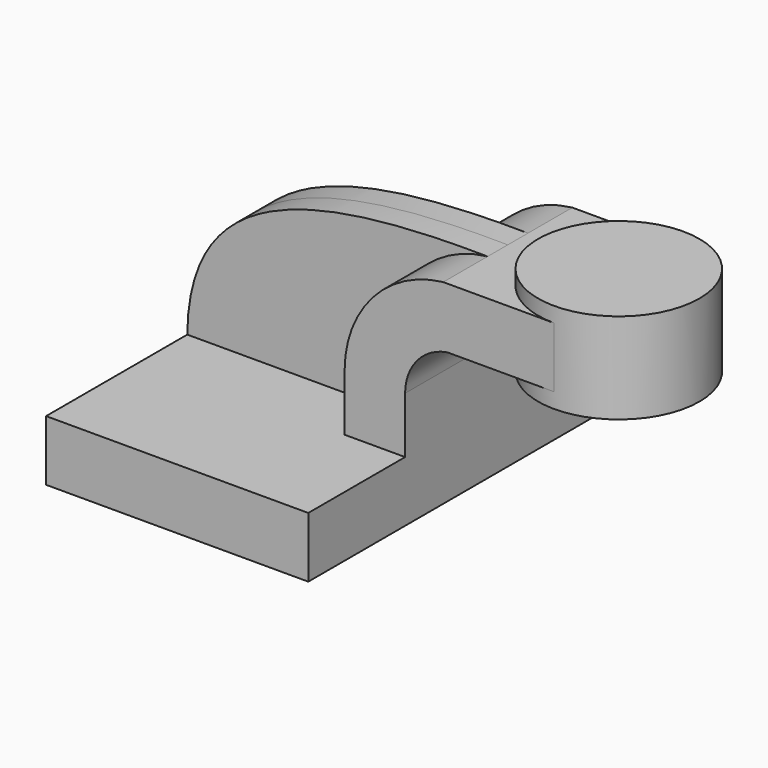
from build123d import *

# Parameters (mm, degrees)
F1_DEPTH = 63.5
F0_W     = 25.4
F0_H     = 19.05
F2_DEPTH = 25.4
F3_DEPTH = 7.9375


with BuildPart() as f1:
    # F0 (on Front) → F1 (new body, symmetric)
    with BuildSketch(Plane.XZ):
        Polygon((-41.275, 9.525), (-41.275, -9.525), (41.275, -9.525), (41.275, 9.525), (22.225, 9.525), align=None)
    extrude(amount=F1_DEPTH, both=True)

    # F0 (on Front) → F2 (join, symmetric)
    with BuildSketch(Plane.XZ):
        with Locations((75.5235318422, 52.4002)):
            Rectangle(F0_W, F0_H)
        with BuildLine():
            Line((22.225, 9.525), (41.275, 9.525))
            Line((41.275, 9.525), (41.275, 27.2153939429))
            ThreePointArc((41.275, 27.2153939429), (45.0386370244, 37.4784593657), (54.5449857479, 42.8752))
            Line((54.5449857479, 42.8752), (62.8235318422, 42.8752))
            Line((62.8235318422, 42.8752), (62.8235318422, 61.9252))
            Line((62.8235318422, 61.9252), (53.2789551181, 61.9252))
            ThreePointArc((53.2789551181, 61.9252), (31.1216321343, 50.5022935057), (22.225, 27.2153939429))
            Line((22.225, 27.2153939429), (22.225, 9.525))
        make_face()
    extrude(amount=F2_DEPTH, both=True)

    # F0 (on Front) → F3 (join, symmetric)
    with BuildSketch(Plane.XZ):
        with BuildLine():
            add(Edge.make_bspline(
                [(-41.275, 9.525), (-40.8366508782, 51.8352910876), (-5.1678125747, 62.6129284501), (53.2789551181, 61.9252)],
                knots=[0, 0, 0, 0, 108.1028740992, 108.1028740992, 108.1028740992, 108.1028740992], degree=3))
            Line((-41.275, 9.525), (22.225, 9.525))
            Line((22.225, 9.525), (22.225, 27.2153939429))
            ThreePointArc((22.225, 27.2153939429), (31.1216321343, 50.5022935057), (53.2789551181, 61.9252))
        make_face()
    extrude(amount=F3_DEPTH, both=True)

    # F0 (on Front) → F4 (revolve)
    with BuildSketch(Plane.XZ):
        Polygon((88.2235318422, 66.675), (88.2235318422, 61.9252), (88.2235318422, 42.8752), (88.2235318422, 38.1), (113.6235318422, 38.1), (113.6235318422, 66.675), align=None)
    revolve(axis=Axis((88.2235318422, 0, 52.3875), (0, 0, 1)))


solid = f1.part
